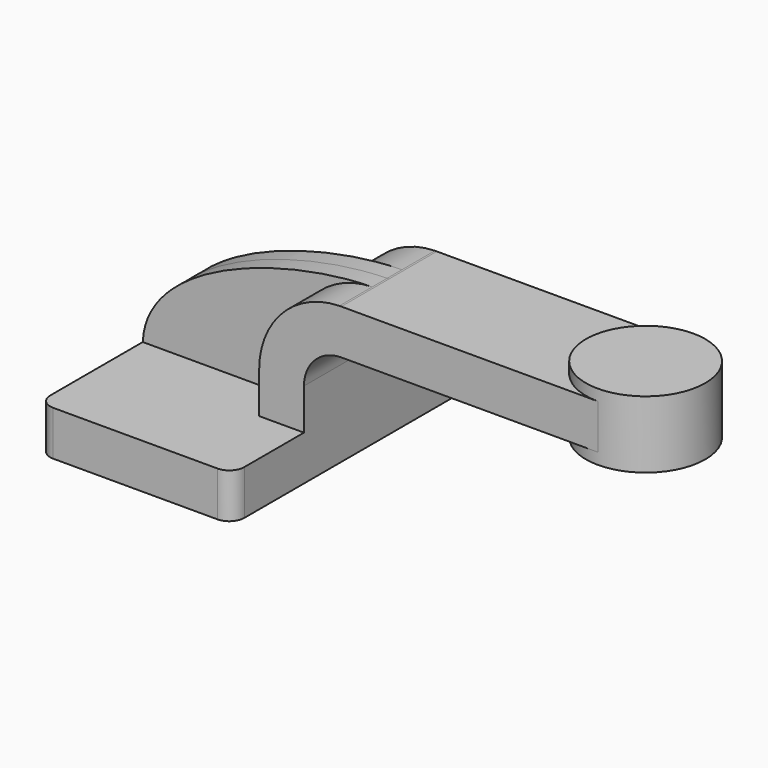
from build123d import *

# Parameters (mm, degrees)
F1_DEPTH = 63.5
F2_DEPTH = 7.9375
F0_W     = 25.4
F0_H     = 19.05
F3_DEPTH = 25.4
F5_R     = 6.35


with BuildPart() as f1:
    # F0 (on Front) → F1 (new body, symmetric)
    with BuildSketch(Plane.XZ):
        Polygon((-41.275, 9.525), (-41.275, -9.525), (41.275, -9.525), (41.275, 9.525), (22.225, 9.525), align=None)
    extrude(amount=F1_DEPTH, both=True)

    # F0 (on Front) → F3 (join, symmetric)
    with BuildSketch(Plane.XZ):
        with BuildLine():
            Line((22.225, 9.525), (41.275, 9.525))
            Line((41.275, 9.525), (41.275, 27.0002))
            ThreePointArc((41.275, 27.0002), (45.9246798487, 38.2255201513), (57.15, 42.8752))
            Line((57.15, 42.8752), (140.9229072666, 42.8752))
            Line((140.9229072666, 42.8752), (140.9229072666, 61.9252))
            Line((140.9229072666, 61.9252), (57.15, 61.9252))
            add(Edge.make_bspline(
                [(56.3476293335, 61.915981909), (56.6162268353, 61.9200045934), (56.8836936428, 61.9230778008), (57.15, 61.9252)],
                knots=[110.7064040288, 110.7064040288, 110.7064040288, 110.7064040288, 111.5045361635, 111.5045361635, 111.5045361635, 111.5045361635], degree=3))
            ThreePointArc((56.3476293335, 61.915981909), (32.1722256743, 51.4105751453), (22.225, 27.0002))
            Line((22.225, 27.0002), (22.225, 9.525))
        make_face()
        with Locations((153.6229072666, 52.4002)):
            Rectangle(F0_W, F0_H)
    extrude(amount=F3_DEPTH, both=True)

    # F0 (on Front) → F4 (revolve)
    with BuildSketch(Plane.XZ):
        Polygon((166.3229072666, 66.675), (166.3229072666, 61.9252), (166.3229072666, 42.8752), (166.3229072666, 38.1), (191.7229072666, 38.1), (191.7229072666, 66.675), align=None)
    revolve(axis=Axis((166.3229072666, 0, 52.3875), (0, 0, -1)))

    # F5
    f5_edges = [f1.edges().sort_by_distance(p)[0] for p in [
        (41.275, -63.5, 0),
        (-41.275, -63.5, 0),
        (-41.275, 63.5, 0),
        (41.275, 63.5, 0),
    ]]
    fillet(f5_edges, radius=F5_R)


with BuildPart() as f2:
    # F0 (on Front) → F2 (new body, symmetric)
    with BuildSketch(Plane.XZ):
        with BuildLine():
            add(Edge.make_bspline(
                [(-41.275, 9.525), (-39.9191045242, 42.5324796176), (19.0913126511, 61.3580079673), (56.3476293335, 61.915981909)],
                knots=[0, 0, 0, 0, 110.7064040288, 110.7064040288, 110.7064040288, 110.7064040288], degree=3))
            Line((-41.275, 9.525), (22.225, 9.525))
            Line((22.225, 9.525), (22.225, 27.0002))
            ThreePointArc((22.225, 27.0002), (32.1722256743, 51.4105751453), (56.3476293335, 61.915981909))
        make_face()
    extrude(amount=F2_DEPTH, both=True)


solid = Compound([f1.part, f2.part])
